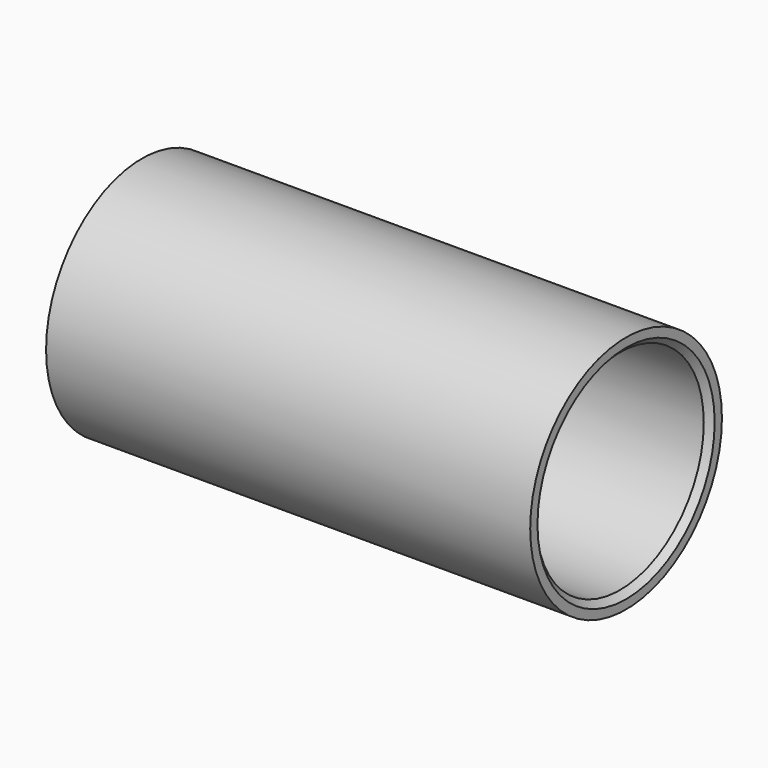
from build123d import *

# Parameters (mm, degrees)
F2_R    = 0.49999
F3_SIZE = 1


# Not quite as in the source:
# - a fillet or chamfer is up to 0.001 mm smaller than in the source, because OpenCascade refuses the exact size


with BuildPart() as f1:
    # F0 (on Top) → F1 (revolve)
    with BuildSketch(Plane.XY):
        Polygon((0, 19.8), (-40, 19.8), (-40, 17.3), (-0.5, 17.3), (-0.5, 16.3), (0, 16.3), (0.5, 16.3), (0.5, 17.3), (40, 17.3), (40, 19.8), align=None)
    revolve(axis=Axis((0, 0, 0), (1, 0, 0)))

    # F2 (radius 0.5 in the source; OpenCascade refuses exactly that, so slightly less here)
    f2_edges = [f1.edges().sort_by_distance(p)[0] for p in [
        (-0.5, -16.3, 0),
        (0.5, -16.3, 0),
    ]]
    fillet(f2_edges, radius=F2_R)

    # F3
    f3_edges = [f1.edges().sort_by_distance(p)[0] for p in [
        (-40, -17.3, 0),
        (40, -17.3, 0),
    ]]
    chamfer(f3_edges, length=F3_SIZE)


solid = f1.part
